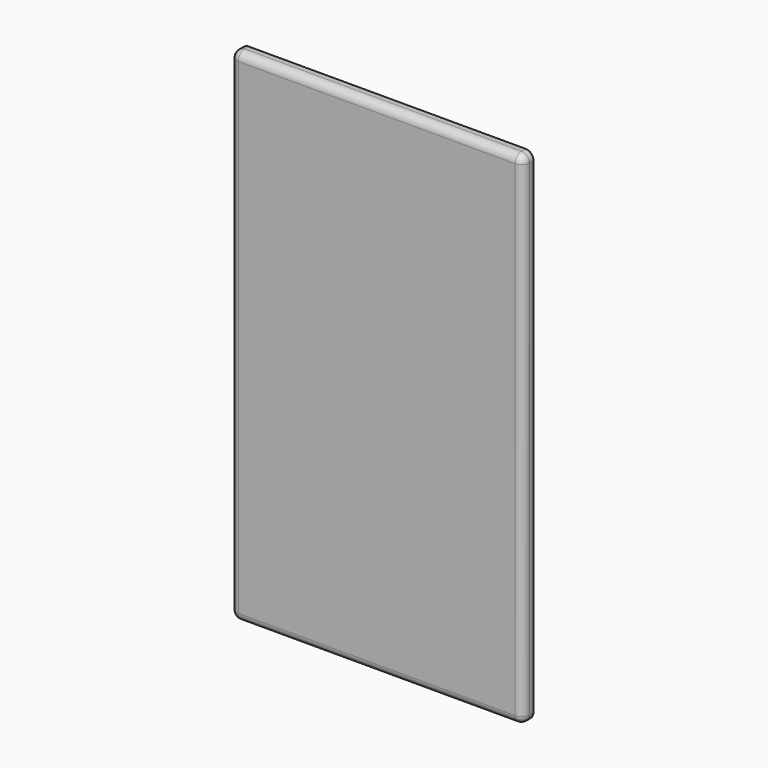
from build123d import *

# Parameters (mm, degrees)
F0_W         = 560
F0_H         = 960
F2_DEPTH     = 25
F3_R         = 15
F4_T1_DEPTH  = 47.5
F4_S5_W      = 15
F4_S5_H      = 15
F4_T6_DEPTH  = 15
F4_S11_W     = 15
F4_S11_H     = 15
F4_T12_DEPTH = 15
F4_S17_W     = 15
F4_S17_H     = 15
F4_T18_DEPTH = 15
F4_S23_W     = 15
F4_S23_H     = 15
F4_T24_DEPTH = 15


# Not quite as in the source:
# - a fillet or chamfer that OpenCascade refuses, or shapes differently, is made with other operations: its cross-section is extruded or revolved along the edge and cut away or added


with BuildPart() as f2:
    # F0 (on Front) → F2 (new body)
    with BuildSketch(Plane.XZ):
        Rectangle(F0_W, F0_H)
    extrude(amount=-F2_DEPTH)

    # F3
    f3_edges = [f2.edges().sort_by_distance(p)[0] for p in [
        (0, 0, 480),
        (-280, 0, 0),
        (0, 0, -480),
        (280, 0, 0),
    ]]
    fillet(f3_edges, radius=F3_R)

    # F4: fillet of radius 15 on 8 edges, made by hand

    # F4_s2 → F4_t1 (cut)
    with BuildSketch(Plane.XZ.offset(-62.5)):
        with BuildLine():
            ThreePointArc((-280, -465), (-275.6066017178, -475.6066017178), (-265, -480))
            Line((-265, -480), (-280, -480))
            Line((-280, -480), (-280, -465))
        make_face()
        with BuildLine():
            ThreePointArc((280, -465), (275.6066017178, -475.6066017178), (265, -480))
            Line((265, -480), (280, -480))
            Line((280, -480), (280, -465))
        make_face()
        with BuildLine():
            ThreePointArc((-265, 480), (-275.6066017178, 475.6066017178), (-280, 465))
            Line((-280, 465), (-280, 480))
            Line((-280, 480), (-265, 480))
        make_face()
        with BuildLine():
            ThreePointArc((265, 480), (275.6066017178, 475.6066017178), (280, 465))
            Line((280, 465), (280, 480))
            Line((280, 480), (265, 480))
        make_face()
    extrude(amount=F4_T1_DEPTH, mode=Mode.SUBTRACT)


with BuildPart() as f4_tool4:
    # F4_s5 → F4_t6 (new body)
    with BuildSketch(Plane.XY.offset(465)):
        with Locations((272.5, 7.5)):
            Rectangle(F4_S5_W, F4_S5_H)
    extrude(amount=F4_T6_DEPTH)

    # F4_s7 → F4_t8 (revolve, cut)
    with BuildSketch(Plane(origin=(265, 15, 465), x_dir=(-0.7071067812, 0.7071067812, 0), z_dir=(0.7071067812, 0.7071067812, 0))):
        with BuildLine():
            ThreePointArc((0, -15), (15, 0), (0, 15))
            Line((0, 15), (0, -15))
        make_face()
    revolve(axis=Axis((265, 15, 465), (0, 0, 1)), mode=Mode.SUBTRACT)


with BuildPart() as f2_1:
    add(f2.part)

    # F4_t3: cut F4_tool4
    add(f4_tool4.part, mode=Mode.SUBTRACT)


with BuildPart() as f4_tool10:
    # F4_s11 → F4_t12 (new body)
    with BuildSketch(Plane.XY.offset(465)):
        with Locations((-272.5, 7.5)):
            Rectangle(F4_S11_W, F4_S11_H)
    extrude(amount=F4_T12_DEPTH)

    # F4_s13 → F4_t14 (revolve, cut)
    with BuildSketch(Plane(origin=(-265, 15, 465), x_dir=(0.7071067812, 0.7071067812, 0), z_dir=(0.7071067812, -0.7071067812, 0))):
        with BuildLine():
            ThreePointArc((0, -15), (15, 0), (0, 15))
            Line((0, 15), (0, -15))
        make_face()
    revolve(axis=Axis((-265, 15, 465), (0, 0, 1)), mode=Mode.SUBTRACT)


with BuildPart() as f2_2:
    add(f2_1.part)

    # F4_t9: cut F4_tool10
    add(f4_tool10.part, mode=Mode.SUBTRACT)


with BuildPart() as f4_tool16:
    # F4_s17 → F4_t18 (new body)
    with BuildSketch(Plane.YZ.offset(265)):
        with Locations((7.5, -472.5)):
            Rectangle(F4_S17_W, F4_S17_H)
    extrude(amount=F4_T18_DEPTH)

    # F4_s19 → F4_t20 (revolve, cut)
    with BuildSketch(Plane(origin=(265, 15, -465), x_dir=(0, 0.7071067812, 0.7071067812), z_dir=(0, 0.7071067812, -0.7071067812))):
        with BuildLine():
            ThreePointArc((0, -15), (15, 0), (0, 15))
            Line((0, 15), (0, -15))
        make_face()
    revolve(axis=Axis((265, 15, -465), (1, 0, 0)), mode=Mode.SUBTRACT)


with BuildPart() as f2_3:
    add(f2_2.part)

    # F4_t15: cut F4_tool16
    add(f4_tool16.part, mode=Mode.SUBTRACT)


with BuildPart() as f4_tool22:
    # F4_s23 → F4_t24 (new body)
    with BuildSketch(Plane.YZ.offset(-265)):
        with Locations((7.5, -472.5)):
            Rectangle(F4_S23_W, F4_S23_H)
    extrude(amount=-F4_T24_DEPTH)

    # F4_s25 → F4_t26 (revolve, cut)
    with BuildSketch(Plane(origin=(-265, 15, -465), x_dir=(0, 0.7071067812, 0.7071067812), z_dir=(0, -0.7071067812, 0.7071067812))):
        with BuildLine():
            ThreePointArc((0, -15), (15, 0), (0, 15))
            Line((0, 15), (0, -15))
        make_face()
    revolve(axis=Axis((-265, 15, -465), (-1, 0, 0)), mode=Mode.SUBTRACT)


with BuildPart() as f2_4:
    add(f2_3.part)

    # F4_t21: cut F4_tool22
    add(f4_tool22.part, mode=Mode.SUBTRACT)


solid = f2_4.part
